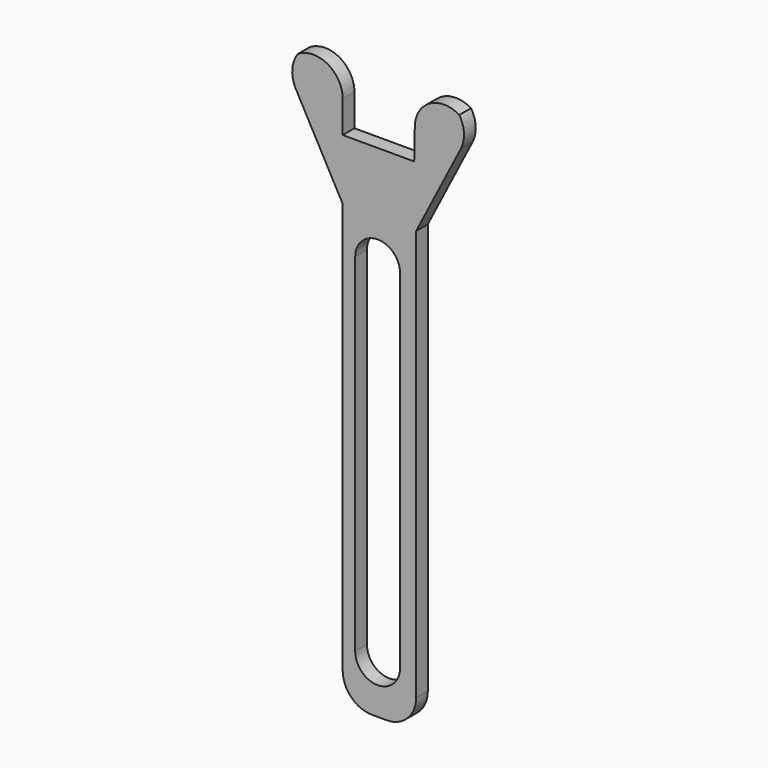
from build123d import *

# Parameters (mm, degrees)
F1_DEPTH    = 2.54
F2_T1_DEPTH = 21.3951912934
F2_T3_DEPTH = 22.4631654102
F2_T5_DEPTH = 27.94
F2_T7_DEPTH = 60.9088837652
F2_T9_DEPTH = 60.1042195061
F4_DEPTH    = 2.541


# Not quite as in the source:
# - a fillet or chamfer that OpenCascade refuses, or shapes differently, is made with other operations: its cross-section is extruded or revolved along the edge and cut away or added


with BuildPart() as f1:
    # F0 (on Front) → F1 (new body)
    with BuildSketch(Plane.XZ):
        Polygon((-49.9376785943, 26.895446232), (-49.9376785943, -49.304553768), (-37.2376785943, -49.304553768), (-37.2376785943, 26.895446232), (-27.7746748179, 45.2916584909), (-37.2376785943, 54.4446781278), (-37.5589355826, 37.401124835), (-49.9376785943, 37.401124835), (-49.9376785943, 54.4446781278), (-59.968046844, 45.2916584909), align=None)
    extrude(amount=F1_DEPTH)

    # F2: fillet of radius 5.08 on 6 edges, made by hand

    # F2_s2 → F2_t1 (cut)
    with BuildSketch(Plane.XZ.offset(-9.4275956467)):
        with BuildLine():
            ThreePointArc((-29.49965362, 41.9382754706), (-29.0047534445, 45.0887624488), (-30.4852273769, 47.9134201836))
            Line((-30.4852273769, 47.9134201836), (-27.7746748179, 45.2916584909))
            Line((-27.7746748179, 45.2916584909), (-29.49965362, 41.9382754706))
        make_face()
    extrude(amount=F2_T1_DEPTH, mode=Mode.SUBTRACT)

    # F2_s4 → F2_t3 (cut)
    with BuildSketch(Plane.XZ.offset(-9.9615827051)):
        with BuildLine():
            ThreePointArc((-57.0247017985, 47.9775514042), (-58.6106651129, 45.064296855), (-58.0605727295, 41.7932526681))
            Line((-58.0605727295, 41.7932526681), (-59.968046844, 45.2916584909))
            Line((-59.968046844, 45.2916584909), (-57.0247017985, 47.9775514042))
        make_face()
    extrude(amount=F2_T3_DEPTH, mode=Mode.SUBTRACT)

    # F2_s6 → F2_t5 (cut)
    with BuildSketch(Plane.XZ.offset(-12.7)):
        with BuildLine():
            ThreePointArc((-42.3176785943, -49.304553768), (-38.7255761459, -47.8166562165), (-37.2376785943, -44.224553768))
            Line((-37.2376785943, -44.224553768), (-37.2376785943, -49.304553768))
            Line((-37.2376785943, -49.304553768), (-42.3176785943, -49.304553768))
        make_face()
        with BuildLine():
            ThreePointArc((-49.9376785943, -44.224553768), (-48.4497810427, -47.8166562165), (-44.8576785943, -49.304553768))
            Line((-44.8576785943, -49.304553768), (-49.9376785943, -49.304553768))
            Line((-49.9376785943, -49.304553768), (-49.9376785943, -44.224553768))
        make_face()
    extrude(amount=F2_T5_DEPTH, mode=Mode.SUBTRACT)

    # F2_s8 → F2_t7 (cut)
    with BuildSketch(Plane.XZ.offset(-29.1844418826)):
        with BuildLine():
            ThreePointArc((-28.8467837584, 46.3286478461), (-34.3174578503, 47.3726785237), (-37.457680624, 42.7729746194))
            Line((-37.457680624, 42.7729746194), (-37.2376785943, 54.4446781278))
            Line((-37.2376785943, 54.4446781278), (-28.8467837584, 46.3286478461))
        make_face()
    extrude(amount=F2_T7_DEPTH, mode=Mode.SUBTRACT)

    # F2_s10 → F2_t9 (cut)
    with BuildSketch(Plane.XZ.offset(-28.782109753)):
        with BuildLine():
            ThreePointArc((-49.9376785943, 42.9318342266), (-52.9669146048, 47.5794967637), (-58.4419175941, 46.6842983866))
            Line((-58.4419175941, 46.6842983866), (-49.9376785943, 54.4446781278))
            Line((-49.9376785943, 54.4446781278), (-49.9376785943, 42.9318342266))
        make_face()
    extrude(amount=F2_T9_DEPTH, mode=Mode.SUBTRACT)

    # F3 (on face) → F4 (cut, through all)
    with BuildSketch(Plane.XZ.offset(2.54)):
        with BuildLine():
            Line((-40.0050021708, -40.580611676), (-40.0050021708, 19.5707920939))
            ThreePointArc((-40.0050021708, 19.5707920939), (-43.8903793693, 23.4561692923), (-47.7757565677, 19.5707920939))
            Line((-47.7757565677, 19.5707920939), (-47.7757565677, -40.580611676))
            ThreePointArc((-47.7757565677, -40.580611676), (-43.8903793693, -44.4659888744), (-40.0050021708, -40.580611676))
        make_face()
    extrude(amount=-F4_DEPTH, mode=Mode.SUBTRACT)


solid = f1.part
